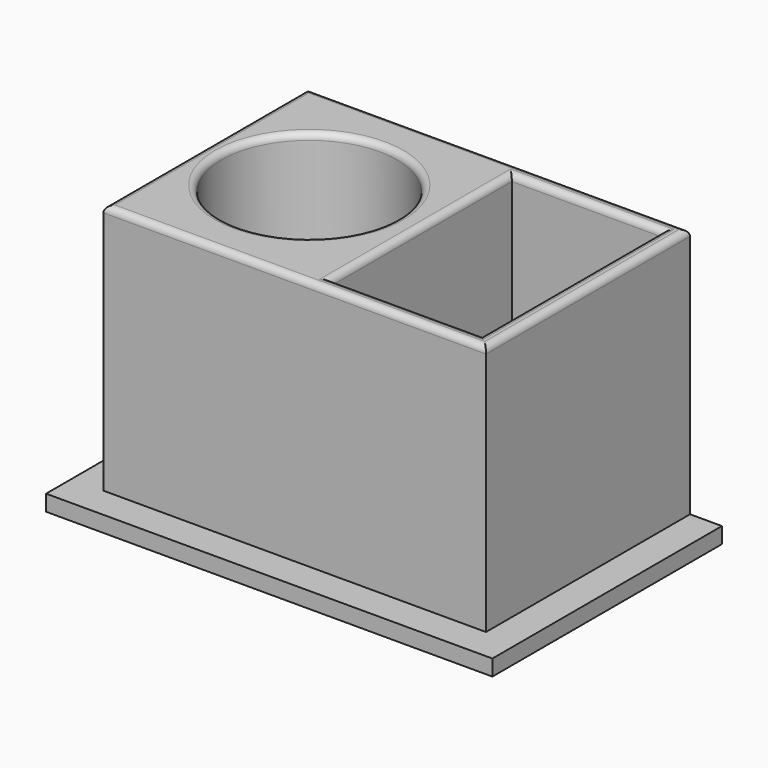
from build123d import *

# Parameters (mm, degrees)
F1_DEPTH = 50
F2_W     = 88.9
F2_H     = 63.5
F2_W_2   = 76.2
F2_H_2   = 50.8
F2_R     = 17.5
F2_W_3   = 30
F2_H_3   = 45
F3_DEPTH = 3.175
F4_W     = 442.8342580795
F4_H     = 256.8548172712
F5_DEPTH = 25.4
F6_R     = 1.27


with BuildPart() as f1:
    # F0 (on Top) → F1 (new body)
    with BuildSketch(Plane.XY):
        Polygon((33.175, -2.9), (33.175, 22.5), (33.175, 47.9), (-43.025, 47.9), (-43.025, 22.5), (-43.025, -2.9), align=None)
        with BuildLine():
            ThreePointArc((-4.85, 22.5), (-22.35, 5), (-39.85, 22.5))
            ThreePointArc((-39.85, 22.5), (-22.35, 40), (-4.85, 22.5))
        make_face(mode=Mode.SUBTRACT)
        Polygon((30, 0), (0, 0), (0, 45), (30, 45), (30, 22.5), align=None, mode=Mode.SUBTRACT)
    extrude(amount=F1_DEPTH)

    # F2 (on face) → F3 (join)
    with BuildSketch(Plane(origin=(0, 0, 0), x_dir=(1, 0, 0), z_dir=(0, 0, -1))):
        with Locations((-4.925, -22.5)):
            Rectangle(F2_W, F2_H)
        with Locations((-4.925, -22.5)):
            Rectangle(F2_W_2, F2_H_2, mode=Mode.SUBTRACT)
        with Locations((-4.925, -22.5)):
            Rectangle(F2_W_2, F2_H_2)
        with Locations((-22.35, -22.5)):
            Circle(F2_R, mode=Mode.SUBTRACT)
        with Locations((15, -22.5)):
            Rectangle(F2_W_3, F2_H_3, mode=Mode.SUBTRACT)
        with Locations((-22.35, -22.5)):
            Circle(F2_R)
        with Locations((15, -22.5)):
            Rectangle(F2_W_3, F2_H_3)
    extrude(amount=F3_DEPTH)

    # F4 (on face) → F5 (cut)
    with BuildSketch(Plane(origin=(0, 47.9, 0), x_dir=(-1, 0, 0), z_dir=(0, 1, 0))):
        with Locations((25.4539847374, 21.782644093)):
            Rectangle(F4_W, F4_H)
    extrude(amount=F5_DEPTH, mode=Mode.SUBTRACT)

    # F6
    f6_edges = [f1.edges().sort_by_distance(p)[0] for p in [
        (0, 22.5, 50),
        (33.175, 22.5, 50),
        (-4.925, 47.9, 50),
        (-43.025, 22.5, 50),
        (-4.925, -2.9, 50),
        (-39.85, 22.5, 50),
        (15, 0, 50),
        (15, 45, 50),
        (30, 22.5, 50),
    ]]
    fillet(f6_edges, radius=F6_R)


solid = f1.part
